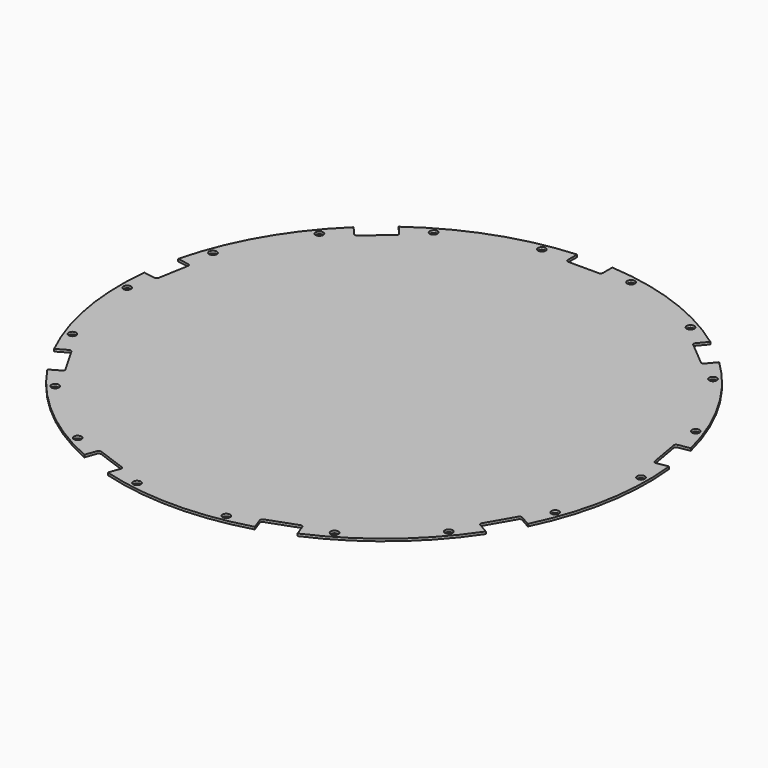
from build123d import *

# Parameters (mm, degrees)
F0_R     = 225
F1_DEPTH = 2
F3_D     = 6.5
F5_DEPTH = 2.001


# Not quite as in the source:
# - a feature names something its author has since deleted; it is built from what else it names


with BuildPart() as f1:
    # F0 (on Top) → F1 (new body)
    with BuildSketch(Plane.XY):
        Circle(F0_R)
    extrude(amount=F1_DEPTH)

    # F3 (through all)
    with Locations(Plane.XY.offset(2)):
        with Locations((219, 0), (205.7926839521, 74.9024113883), (167.7637330431, 140.7704865214), (109.5, 189.6595634288), (38.0289509091, 215.6728979097), (-38.0289509091, 215.6728979097), (-109.5, 189.6595634288), (-167.7637330431, 140.7704865214), (-205.7926839521, 74.9024113883), (-219, 0), (-205.7926839521, -74.9024113883), (-167.7637330431, -140.7704865214), (-109.5, -189.6595634288), (-38.0289509091, -215.6728979097), (38.0289509091, -215.6728979097), (109.5, -189.6595634288), (167.7637330431, -140.7704865214), (205.7926839521, -74.9024113883)):
            Hole(F3_D / 2)

    # F4 (on face) → F5 (cut, through all)
    with BuildSketch(Plane.XY.offset(2)):
        with BuildLine():
            ThreePointArc((223.6935148816, 24.2118029049), (221.5817444277, 39.0708399751), (218.4840695516, 53.7560354952))
            Line((218.4840695516, 53.7560354952), (208.6359920215, 52.0195537186))
            ThreePointArc((208.6359920215, 52.0195537186), (207.3449842883, 51.1970910852), (207.0136728708, 49.7026418572))
            Line((207.0136728708, 49.7026418572), (209.2710991805, 36.900141068))
            Line((209.2710991805, 36.900141068), (211.5285254901, 24.0976402789))
            ThreePointArc((211.5285254901, 24.0976402789), (212.3509881235, 22.8066325456), (213.8454373515, 22.4753211282))
            Line((213.8454373515, 22.4753211282), (223.6935148816, 24.2118029049))
        make_face()
        with BuildLine():
            Line((149.3682510245, 154.6742923751), (155.7961271214, 162.3347368063))
            ThreePointArc((155.7961271214, 162.3347368063), (144.6272121795, 172.3599997018), (132.8147938278, 181.6183650969))
            Line((132.8147938278, 181.6183650969), (126.386917731, 173.9579206657))
            ThreePointArc((126.386917731, 173.9579206657), (125.926617221, 172.4980339608), (126.6334313978, 171.1402565601))
            Line((126.6334313978, 171.1402565601), (136.5920091584, 162.7840176342))
            Line((136.5920091584, 162.7840176342), (146.5505869189, 154.4277787082))
            ThreePointArc((146.5505869189, 154.4277787082), (148.0104736238, 153.9674781983), (149.3682510245, 154.6742923751))
        make_face()
        with BuildLine():
            Line((15, 214.4994432064), (15, 224.4994432064))
            ThreePointArc((15, 224.4994432064), (0, 225), (-15, 224.4994432064))
            Line((-15, 224.4994432064), (-15, 214.4994432064))
            ThreePointArc((-15, 214.4994432064), (-14.4142135624, 213.0852296441), (-13, 212.4994432064))
            Line((-13, 212.4994432064), (0, 212.4994432064))
            Line((0, 212.4994432064), (13, 212.4994432064))
            ThreePointArc((13, 212.4994432064), (14.4142135624, 213.0852296441), (15, 214.4994432064))
        make_face()
        with BuildLine():
            Line((-126.386917731, 173.9579206657), (-132.8147938278, 181.6183650969))
            ThreePointArc((-132.8147938278, 181.6183650969), (-144.6272121795, 172.3599997018), (-155.7961271214, 162.3347368063))
            Line((-155.7961271214, 162.3347368063), (-149.3682510245, 154.6742923751))
            ThreePointArc((-149.3682510245, 154.6742923751), (-148.0104736238, 153.9674781983), (-146.5505869189, 154.4277787082))
            Line((-146.5505869189, 154.4277787082), (-136.5920091584, 162.7840176342))
            Line((-136.5920091584, 162.7840176342), (-126.6334313978, 171.1402565601))
            ThreePointArc((-126.6334313978, 171.1402565601), (-125.926617221, 172.4980339608), (-126.386917731, 173.9579206657))
        make_face()
        with BuildLine():
            Line((-208.6359920215, 52.0195537186), (-218.4840695516, 53.7560354952))
            ThreePointArc((-218.4840695516, 53.7560354952), (-221.5817444277, 39.0708399751), (-223.6935148816, 24.2118029049))
            Line((-223.6935148816, 24.2118029049), (-213.8454373515, 22.4753211282))
            ThreePointArc((-213.8454373515, 22.4753211282), (-212.3509881235, 22.8066325456), (-211.5285254901, 24.0976402789))
            Line((-211.5285254901, 24.0976402789), (-209.2710991805, 36.900141068))
            Line((-209.2710991805, 36.900141068), (-207.0136728708, 49.7026418572))
            ThreePointArc((-207.0136728708, 49.7026418572), (-207.3449842883, 51.1970910852), (-208.6359920215, 52.0195537186))
        make_face()
        with BuildLine():
            ThreePointArc((-201.9222209522, -99.2593405465), (-194.8557158515, -112.5), (-186.9222209522, -125.24010266))
            Line((-186.9222209522, -125.24010266), (-178.2619669144, -120.24010266))
            ThreePointArc((-178.2619669144, -120.24010266), (-177.3301152618, -119.0256899426), (-177.5299161068, -117.5080518524))
            Line((-177.5299161068, -117.5080518524), (-184.0299161068, -106.2497216032))
            Line((-184.0299161068, -106.2497216032), (-190.5299161068, -94.991391354))
            ThreePointArc((-190.5299161068, -94.991391354), (-191.7443288242, -94.0595397014), (-193.2619669144, -94.2593405465))
            Line((-193.2619669144, -94.2593405465), (-201.9222209522, -99.2593405465))
        make_face()
        with BuildLine():
            ThreePointArc((-90.8787210538, -205.8301680017), (-76.9545322483, -211.4308396768), (-62.6879424302, -216.0907723015))
            Line((-62.6879424302, -216.0907723015), (-59.267740997, -206.6938460937))
            ThreePointArc((-59.267740997, -206.6938460937), (-59.3345106645, -205.1645692835), (-60.4630859519, -204.1304205654))
            Line((-60.4630859519, -204.1304205654), (-72.6790900221, -199.6841587022))
            Line((-72.6790900221, -199.6841587022), (-84.8950940923, -195.237896839))
            ThreePointArc((-84.8950940923, -195.237896839), (-86.4243709024, -195.3046665065), (-87.4585196205, -196.4332417939))
            Line((-87.4585196205, -196.4332417939), (-90.8787210538, -205.8301680017))
        make_face()
        with BuildLine():
            ThreePointArc((62.6879424302, -216.0907723015), (76.9545322483, -211.4308396768), (90.8787210538, -205.8301680017))
            Line((90.8787210538, -205.8301680017), (87.4585196205, -196.4332417939))
            ThreePointArc((87.4585196205, -196.4332417939), (86.4243709024, -195.3046665065), (84.8950940923, -195.237896839))
            Line((84.8950940923, -195.237896839), (72.6790900221, -199.6841587022))
            Line((72.6790900221, -199.6841587022), (60.4630859519, -204.1304205654))
            ThreePointArc((60.4630859519, -204.1304205654), (59.3345106645, -205.1645692835), (59.267740997, -206.6938460937))
            Line((59.267740997, -206.6938460937), (62.6879424302, -216.0907723015))
        make_face()
        with BuildLine():
            ThreePointArc((186.9222209522, -125.24010266), (194.8557158515, -112.5), (201.9222209522, -99.2593405465))
            Line((201.9222209522, -99.2593405465), (193.2619669144, -94.2593405465))
            ThreePointArc((193.2619669144, -94.2593405465), (191.7443288242, -94.0595397014), (190.5299161068, -94.991391354))
            Line((190.5299161068, -94.991391354), (184.0299161068, -106.2497216032))
            Line((184.0299161068, -106.2497216032), (177.5299161068, -117.5080518524))
            ThreePointArc((177.5299161068, -117.5080518524), (177.3301152618, -119.0256899426), (178.2619669144, -120.24010266))
            Line((178.2619669144, -120.24010266), (186.9222209522, -125.24010266))
        make_face()
    extrude(amount=-F5_DEPTH, mode=Mode.SUBTRACT)


solid = f1.part
